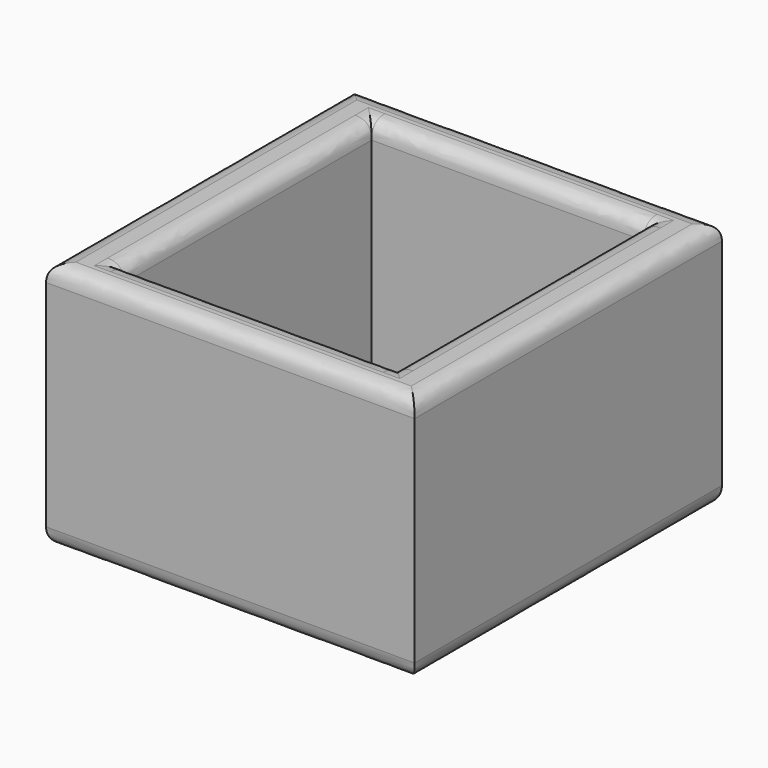
from build123d import *

# Parameters (mm, degrees)
F0_W         = 113.1491363049
F0_H         = 117.9769933224
F1_DEPTH     = 76.2
F2_W         = 83.599075675
F2_H         = 95.0139909983
F3_DEPTH     = 105.1160246134
F4_T1_DEPTH  = 83.599075675
F4_T3_DEPTH  = 95.0139909983
F4_T5_DEPTH  = 138.5491363049
F4_T7_DEPTH  = 143.3769933224
F4_T13_DEPTH = 96.299075675
F4_T17_DEPTH = 107.7139909983
F4_T24_DEPTH = 107.7139909983
F4_T28_DEPTH = 96.299075675
F4_T35_DEPTH = 107.7139909983
F4_T39_DEPTH = 96.299075675
F4_T46_DEPTH = 107.7139909983
F4_T50_DEPTH = 96.299075675
F4_T57_DEPTH = 96.299075675
F4_T61_DEPTH = 107.7139909983
F4_T68_DEPTH = 96.299075675
F4_T72_DEPTH = 107.7139909983
F4_T79_DEPTH = 107.7139909983
F4_T83_DEPTH = 96.299075675
F4_T90_DEPTH = 96.299075675
F4_T94_DEPTH = 107.7139909983


# Not quite as in the source:
# - a fillet or chamfer that OpenCascade refuses, or shapes differently, is made with other operations: its cross-section is extruded or revolved along the edge and cut away or added


with BuildPart() as f1:
    # F0 (on Top) → F1 (new body)
    with BuildSketch(Plane.XY):
        Rectangle(F0_W, F0_H)
    extrude(amount=F1_DEPTH)

    # F2 (on Top) → F3 (cut)
    with BuildSketch(Plane.XY):
        Rectangle(F2_W, F2_H)
    extrude(amount=F3_DEPTH, mode=Mode.SUBTRACT)

    # F4: fillet of radius 5.08 on 16 edges, made by hand

    # F4_s2 → F4_t1 (cut)
    with BuildSketch(Plane.YZ.offset(-41.7995378375)):
        with BuildLine():
            add(Edge.make_bspline(
                [(-52.5869954991, 76.2), (-47.5069954991, 76.2), (-47.5069954991, 71.12)],
                knots=[0, 0, 0, 1, 1, 1], degree=2, weights=[1, 1, 1]))
            Line((-47.5069954991, 71.12), (-47.5069954991, 76.2))
            Line((-47.5069954991, 76.2), (-52.5869954991, 76.2))
        make_face()
        with BuildLine():
            add(Edge.make_bspline(
                [(52.5869954991, 76.2), (47.5069954991, 76.2), (47.5069954991, 71.12)],
                knots=[0, 0, 0, 1, 1, 1], degree=2, weights=[1, 1, 1]))
            Line((47.5069954991, 71.12), (47.5069954991, 76.2))
            Line((47.5069954991, 76.2), (52.5869954991, 76.2))
        make_face()
        with BuildLine():
            add(Edge.make_bspline(
                [(52.5869954991, 0), (47.5069954991, 0), (47.5069954991, 5.08)],
                knots=[0, 0, 0, 1, 1, 1], degree=2, weights=[1, 1, 1]))
            Line((47.5069954991, 5.08), (47.5069954991, 0))
            Line((47.5069954991, 0), (52.5869954991, 0))
        make_face()
        with BuildLine():
            add(Edge.make_bspline(
                [(-52.5869954991, 0), (-47.5069954991, 0), (-47.5069954991, 5.08)],
                knots=[0, 0, 0, 1, 1, 1], degree=2, weights=[1, 1, 1]))
            Line((-47.5069954991, 5.08), (-47.5069954991, 0))
            Line((-47.5069954991, 0), (-52.5869954991, 0))
        make_face()
    extrude(amount=F4_T1_DEPTH, mode=Mode.SUBTRACT)

    # F4_s4 → F4_t3 (cut)
    with BuildSketch(Plane.XZ.offset(-47.5069954991)):
        with BuildLine():
            add(Edge.make_bspline(
                [(-46.8795378375, 76.2), (-41.7995378375, 76.2), (-41.7995378375, 71.12)],
                knots=[0, 0, 0, 1, 1, 1], degree=2, weights=[1, 1, 1]))
            Line((-41.7995378375, 71.12), (-41.7995378375, 76.2))
            Line((-41.7995378375, 76.2), (-46.8795378375, 76.2))
        make_face()
        with BuildLine():
            add(Edge.make_bspline(
                [(46.8795378375, 76.2), (41.7995378375, 76.2), (41.7995378375, 71.12)],
                knots=[0, 0, 0, 1, 1, 1], degree=2, weights=[1, 1, 1]))
            Line((41.7995378375, 71.12), (41.7995378375, 76.2))
            Line((41.7995378375, 76.2), (46.8795378375, 76.2))
        make_face()
        with BuildLine():
            add(Edge.make_bspline(
                [(-46.8795378375, 0), (-41.7995378375, 0), (-41.7995378375, 5.08)],
                knots=[0, 0, 0, 1, 1, 1], degree=2, weights=[1, 1, 1]))
            Line((-41.7995378375, 5.08), (-41.7995378375, 0))
            Line((-41.7995378375, 0), (-46.8795378375, 0))
        make_face()
        with BuildLine():
            add(Edge.make_bspline(
                [(46.8795378375, 0), (41.7995378375, 0), (41.7995378375, 5.08)],
                knots=[0, 0, 0, 1, 1, 1], degree=2, weights=[1, 1, 1]))
            Line((41.7995378375, 5.08), (41.7995378375, 0))
            Line((41.7995378375, 0), (46.8795378375, 0))
        make_face()
    extrude(amount=F4_T3_DEPTH, mode=Mode.SUBTRACT)

    # F4_s6 → F4_t5 (cut)
    with BuildSketch(Plane.YZ.offset(-69.2745681524)):
        with BuildLine():
            add(Edge.make_bspline(
                [(53.9084966612, 76.2), (58.9884966612, 76.2), (58.9884966612, 71.12)],
                knots=[0, 0, 0, 1, 1, 1], degree=2, weights=[1, 1, 1]))
            Line((58.9884966612, 71.12), (58.9884966612, 76.2))
            Line((58.9884966612, 76.2), (53.9084966612, 76.2))
        make_face()
        with BuildLine():
            add(Edge.make_bspline(
                [(-58.9884966612, 71.12), (-58.9884966612, 76.2), (-53.9084966612, 76.2)],
                knots=[0, 0, 0, 1, 1, 1], degree=2, weights=[1, 1, 1]))
            Line((-53.9084966612, 76.2), (-58.9884966612, 76.2))
            Line((-58.9884966612, 76.2), (-58.9884966612, 71.12))
        make_face()
        with BuildLine():
            add(Edge.make_bspline(
                [(-58.9884966612, 5.08), (-58.9884966612, 0), (-53.9084966612, 0)],
                knots=[0, 0, 0, 1, 1, 1], degree=2, weights=[1, 1, 1]))
            Line((-53.9084966612, 0), (-58.9884966612, 0))
            Line((-58.9884966612, 0), (-58.9884966612, 5.08))
        make_face()
        with BuildLine():
            add(Edge.make_bspline(
                [(53.9084966612, 0), (58.9884966612, 0), (58.9884966612, 5.08)],
                knots=[0, 0, 0, 1, 1, 1], degree=2, weights=[1, 1, 1]))
            Line((58.9884966612, 5.08), (58.9884966612, 0))
            Line((58.9884966612, 0), (53.9084966612, 0))
        make_face()
    extrude(amount=F4_T5_DEPTH, mode=Mode.SUBTRACT)

    # F4_s8 → F4_t7 (cut)
    with BuildSketch(Plane.XZ.offset(-71.6884966612)):
        with BuildLine():
            add(Edge.make_bspline(
                [(56.5745681524, 71.12), (56.5745681524, 76.2), (51.4945681524, 76.2)],
                knots=[0, 0, 0, 1, 1, 1], degree=2, weights=[1, 1, 1]))
            Line((51.4945681524, 76.2), (56.5745681524, 76.2))
            Line((56.5745681524, 76.2), (56.5745681524, 71.12))
        make_face()
        with BuildLine():
            add(Edge.make_bspline(
                [(-56.5745681524, 71.12), (-56.5745681524, 76.2), (-51.4945681524, 76.2)],
                knots=[0, 0, 0, 1, 1, 1], degree=2, weights=[1, 1, 1]))
            Line((-51.4945681524, 76.2), (-56.5745681524, 76.2))
            Line((-56.5745681524, 76.2), (-56.5745681524, 71.12))
        make_face()
        with BuildLine():
            add(Edge.make_bspline(
                [(-56.5745681524, 5.08), (-56.5745681524, 0), (-51.4945681524, 0)],
                knots=[0, 0, 0, 1, 1, 1], degree=2, weights=[1, 1, 1]))
            Line((-51.4945681524, 0), (-56.5745681524, 0))
            Line((-56.5745681524, 0), (-56.5745681524, 5.08))
        make_face()
        with BuildLine():
            add(Edge.make_bspline(
                [(56.5745681524, 5.08), (56.5745681524, 0), (51.4945681524, 0)],
                knots=[0, 0, 0, 1, 1, 1], degree=2, weights=[1, 1, 1]))
            Line((51.4945681524, 0), (56.5745681524, 0))
            Line((56.5745681524, 0), (56.5745681524, 5.08))
        make_face()
    extrude(amount=F4_T7_DEPTH, mode=Mode.SUBTRACT)


with BuildPart() as f4_tool11:
    # F4_s12 → F4_t13 (new body)
    with BuildSketch(Plane.YZ.offset(54.4995378375)):
        with BuildLine():
            add(Edge.make_bspline(
                [(-52.5869954991, 76.2), (-47.5069954991, 76.2), (-47.5069954991, 71.12)],
                knots=[0, 0, 0, 1, 1, 1], degree=2, weights=[1, 1, 1]))
            Line((-47.5069954991, 71.12), (-47.5069954991, 76.2))
            Line((-47.5069954991, 76.2), (-52.5869954991, 76.2))
        make_face()
    extrude(amount=-F4_T13_DEPTH)

    split(bisect_by=Plane.YZ.offset(41.7995378375), keep=Keep.TOP)


with BuildPart() as f4_tool15:
    # F4_s16 → F4_t17 (new body)
    with BuildSketch(Plane.XZ.offset(-47.5069954991)):
        with BuildLine():
            add(Edge.make_bspline(
                [(46.8795378375, 76.2), (41.7995378375, 76.2), (41.7995378375, 71.12)],
                knots=[0, 0, 0, 1, 1, 1], degree=2, weights=[1, 1, 1]))
            Line((41.7995378375, 71.12), (41.7995378375, 76.2))
            Line((41.7995378375, 76.2), (46.8795378375, 76.2))
        make_face()
    extrude(amount=F4_T17_DEPTH)

    split(bisect_by=Plane.XZ.offset(47.5069954991), keep=Keep.TOP)


with BuildPart() as f4_tool11_1:
    add(f4_tool11.part)

    # F4_t19: intersect F4_tool15
    add(f4_tool15.part, mode=Mode.INTERSECT)


with BuildPart() as f1_1:
    add(f1.part)

    # F4_t9: cut F4_tool11
    add(f4_tool11_1.part, mode=Mode.SUBTRACT)


with BuildPart() as f4_tool22:
    # F4_s23 → F4_t24 (new body)
    with BuildSketch(Plane.XZ.offset(60.2069954991)):
        with BuildLine():
            add(Edge.make_bspline(
                [(-46.8795378375, 76.2), (-41.7995378375, 76.2), (-41.7995378375, 71.12)],
                knots=[0, 0, 0, 1, 1, 1], degree=2, weights=[1, 1, 1]))
            Line((-41.7995378375, 71.12), (-41.7995378375, 76.2))
            Line((-41.7995378375, 76.2), (-46.8795378375, 76.2))
        make_face()
    extrude(amount=-F4_T24_DEPTH)

    split(bisect_by=Plane.XZ.offset(47.5069954991), keep=Keep.TOP)


with BuildPart() as f4_tool26:
    # F4_s27 → F4_t28 (new body)
    with BuildSketch(Plane.YZ.offset(41.7995378375)):
        with BuildLine():
            add(Edge.make_bspline(
                [(-52.5869954991, 76.2), (-47.5069954991, 76.2), (-47.5069954991, 71.12)],
                knots=[0, 0, 0, 1, 1, 1], degree=2, weights=[1, 1, 1]))
            Line((-47.5069954991, 71.12), (-47.5069954991, 76.2))
            Line((-47.5069954991, 76.2), (-52.5869954991, 76.2))
        make_face()
    extrude(amount=-F4_T28_DEPTH)

    split(bisect_by=Plane.YZ.offset(-41.7995378375), keep=Keep.BOTTOM)


with BuildPart() as f4_tool22_1:
    add(f4_tool22.part)

    # F4_t30: intersect F4_tool26
    add(f4_tool26.part, mode=Mode.INTERSECT)


with BuildPart() as f1_2:
    add(f1_1.part)

    # F4_t20: cut F4_tool22
    add(f4_tool22_1.part, mode=Mode.SUBTRACT)


with BuildPart() as f4_tool33:
    # F4_s34 → F4_t35 (new body)
    with BuildSketch(Plane.XZ.offset(47.5069954991)):
        with BuildLine():
            add(Edge.make_bspline(
                [(-46.8795378375, 76.2), (-41.7995378375, 76.2), (-41.7995378375, 71.12)],
                knots=[0, 0, 0, 1, 1, 1], degree=2, weights=[1, 1, 1]))
            Line((-41.7995378375, 71.12), (-41.7995378375, 76.2))
            Line((-41.7995378375, 76.2), (-46.8795378375, 76.2))
        make_face()
    extrude(amount=-F4_T35_DEPTH)

    split(bisect_by=Plane.XZ.offset(-47.5069954991), keep=Keep.BOTTOM)


with BuildPart() as f4_tool37:
    # F4_s38 → F4_t39 (new body)
    with BuildSketch(Plane.YZ.offset(-54.4995378375)):
        with BuildLine():
            add(Edge.make_bspline(
                [(52.5869954991, 76.2), (47.5069954991, 76.2), (47.5069954991, 71.12)],
                knots=[0, 0, 0, 1, 1, 1], degree=2, weights=[1, 1, 1]))
            Line((47.5069954991, 71.12), (47.5069954991, 76.2))
            Line((47.5069954991, 76.2), (52.5869954991, 76.2))
        make_face()
    extrude(amount=F4_T39_DEPTH)

    split(bisect_by=Plane.YZ.offset(-41.7995378375), keep=Keep.BOTTOM)


with BuildPart() as f4_tool33_1:
    add(f4_tool33.part)

    # F4_t41: intersect F4_tool37
    add(f4_tool37.part, mode=Mode.INTERSECT)


with BuildPart() as f1_3:
    add(f1_2.part)

    # F4_t31: cut F4_tool33
    add(f4_tool33_1.part, mode=Mode.SUBTRACT)


with BuildPart() as f4_tool44:
    # F4_s45 → F4_t46 (new body)
    with BuildSketch(Plane.XZ.offset(-60.2069954991)):
        with BuildLine():
            add(Edge.make_bspline(
                [(46.8795378375, 76.2), (41.7995378375, 76.2), (41.7995378375, 71.12)],
                knots=[0, 0, 0, 1, 1, 1], degree=2, weights=[1, 1, 1]))
            Line((41.7995378375, 71.12), (41.7995378375, 76.2))
            Line((41.7995378375, 76.2), (46.8795378375, 76.2))
        make_face()
    extrude(amount=F4_T46_DEPTH)

    split(bisect_by=Plane.XZ.offset(-47.5069954991), keep=Keep.BOTTOM)


with BuildPart() as f4_tool48:
    # F4_s49 → F4_t50 (new body)
    with BuildSketch(Plane.YZ.offset(-41.7995378375)):
        with BuildLine():
            add(Edge.make_bspline(
                [(52.5869954991, 76.2), (47.5069954991, 76.2), (47.5069954991, 71.12)],
                knots=[0, 0, 0, 1, 1, 1], degree=2, weights=[1, 1, 1]))
            Line((47.5069954991, 71.12), (47.5069954991, 76.2))
            Line((47.5069954991, 76.2), (52.5869954991, 76.2))
        make_face()
    extrude(amount=F4_T50_DEPTH)

    split(bisect_by=Plane.YZ.offset(41.7995378375), keep=Keep.TOP)


with BuildPart() as f4_tool44_1:
    add(f4_tool44.part)

    # F4_t52: intersect F4_tool48
    add(f4_tool48.part, mode=Mode.INTERSECT)


with BuildPart() as f1_4:
    add(f1_3.part)

    # F4_t42: cut F4_tool44
    add(f4_tool44_1.part, mode=Mode.SUBTRACT)


with BuildPart() as f4_tool55:
    # F4_s56 → F4_t57 (new body)
    with BuildSketch(Plane.YZ.offset(54.4995378375)):
        with BuildLine():
            add(Edge.make_bspline(
                [(52.5869954991, 0), (47.5069954991, 0), (47.5069954991, 5.08)],
                knots=[0, 0, 0, 1, 1, 1], degree=2, weights=[1, 1, 1]))
            Line((47.5069954991, 5.08), (47.5069954991, 0))
            Line((47.5069954991, 0), (52.5869954991, 0))
        make_face()
    extrude(amount=-F4_T57_DEPTH)

    split(bisect_by=Plane.YZ.offset(41.7995378375), keep=Keep.TOP)


with BuildPart() as f4_tool59:
    # F4_s60 → F4_t61 (new body)
    with BuildSketch(Plane.XZ.offset(47.5069954991)):
        with BuildLine():
            add(Edge.make_bspline(
                [(46.8795378375, 0), (41.7995378375, 0), (41.7995378375, 5.08)],
                knots=[0, 0, 0, 1, 1, 1], degree=2, weights=[1, 1, 1]))
            Line((41.7995378375, 5.08), (41.7995378375, 0))
            Line((41.7995378375, 0), (46.8795378375, 0))
        make_face()
    extrude(amount=-F4_T61_DEPTH)

    split(bisect_by=Plane.XZ.offset(-47.5069954991), keep=Keep.BOTTOM)


with BuildPart() as f4_tool55_1:
    add(f4_tool55.part)

    # F4_t63: intersect F4_tool59
    add(f4_tool59.part, mode=Mode.INTERSECT)


with BuildPart() as f1_5:
    add(f1_4.part)

    # F4_t53: cut F4_tool55
    add(f4_tool55_1.part, mode=Mode.SUBTRACT)


with BuildPart() as f4_tool66:
    # F4_s67 → F4_t68 (new body)
    with BuildSketch(Plane.YZ.offset(41.7995378375)):
        with BuildLine():
            add(Edge.make_bspline(
                [(52.5869954991, 0), (47.5069954991, 0), (47.5069954991, 5.08)],
                knots=[0, 0, 0, 1, 1, 1], degree=2, weights=[1, 1, 1]))
            Line((47.5069954991, 5.08), (47.5069954991, 0))
            Line((47.5069954991, 0), (52.5869954991, 0))
        make_face()
    extrude(amount=-F4_T68_DEPTH)

    split(bisect_by=Plane.YZ.offset(-41.7995378375), keep=Keep.BOTTOM)


with BuildPart() as f4_tool70:
    # F4_s71 → F4_t72 (new body)
    with BuildSketch(Plane.XZ.offset(-60.2069954991)):
        with BuildLine():
            add(Edge.make_bspline(
                [(-46.8795378375, 0), (-41.7995378375, 0), (-41.7995378375, 5.08)],
                knots=[0, 0, 0, 1, 1, 1], degree=2, weights=[1, 1, 1]))
            Line((-41.7995378375, 5.08), (-41.7995378375, 0))
            Line((-41.7995378375, 0), (-46.8795378375, 0))
        make_face()
    extrude(amount=F4_T72_DEPTH)

    split(bisect_by=Plane.XZ.offset(-47.5069954991), keep=Keep.BOTTOM)


with BuildPart() as f4_tool66_1:
    add(f4_tool66.part)

    # F4_t74: intersect F4_tool70
    add(f4_tool70.part, mode=Mode.INTERSECT)


with BuildPart() as f1_6:
    add(f1_5.part)

    # F4_t64: cut F4_tool66
    add(f4_tool66_1.part, mode=Mode.SUBTRACT)


with BuildPart() as f4_tool77:
    # F4_s78 → F4_t79 (new body)
    with BuildSketch(Plane.XZ.offset(-47.5069954991)):
        with BuildLine():
            add(Edge.make_bspline(
                [(-46.8795378375, 0), (-41.7995378375, 0), (-41.7995378375, 5.08)],
                knots=[0, 0, 0, 1, 1, 1], degree=2, weights=[1, 1, 1]))
            Line((-41.7995378375, 5.08), (-41.7995378375, 0))
            Line((-41.7995378375, 0), (-46.8795378375, 0))
        make_face()
    extrude(amount=F4_T79_DEPTH)

    split(bisect_by=Plane.XZ.offset(47.5069954991), keep=Keep.TOP)


with BuildPart() as f4_tool81:
    # F4_s82 → F4_t83 (new body)
    with BuildSketch(Plane.YZ.offset(-54.4995378375)):
        with BuildLine():
            add(Edge.make_bspline(
                [(-52.5869954991, 0), (-47.5069954991, 0), (-47.5069954991, 5.08)],
                knots=[0, 0, 0, 1, 1, 1], degree=2, weights=[1, 1, 1]))
            Line((-47.5069954991, 5.08), (-47.5069954991, 0))
            Line((-47.5069954991, 0), (-52.5869954991, 0))
        make_face()
    extrude(amount=F4_T83_DEPTH)

    split(bisect_by=Plane.YZ.offset(-41.7995378375), keep=Keep.BOTTOM)


with BuildPart() as f4_tool77_1:
    add(f4_tool77.part)

    # F4_t85: intersect F4_tool81
    add(f4_tool81.part, mode=Mode.INTERSECT)


with BuildPart() as f1_7:
    add(f1_6.part)

    # F4_t75: cut F4_tool77
    add(f4_tool77_1.part, mode=Mode.SUBTRACT)


with BuildPart() as f4_tool88:
    # F4_s89 → F4_t90 (new body)
    with BuildSketch(Plane.YZ.offset(-41.7995378375)):
        with BuildLine():
            add(Edge.make_bspline(
                [(-52.5869954991, 0), (-47.5069954991, 0), (-47.5069954991, 5.08)],
                knots=[0, 0, 0, 1, 1, 1], degree=2, weights=[1, 1, 1]))
            Line((-47.5069954991, 5.08), (-47.5069954991, 0))
            Line((-47.5069954991, 0), (-52.5869954991, 0))
        make_face()
    extrude(amount=F4_T90_DEPTH)

    split(bisect_by=Plane.YZ.offset(41.7995378375), keep=Keep.TOP)


with BuildPart() as f4_tool92:
    # F4_s93 → F4_t94 (new body)
    with BuildSketch(Plane.XZ.offset(60.2069954991)):
        with BuildLine():
            add(Edge.make_bspline(
                [(46.8795378375, 0), (41.7995378375, 0), (41.7995378375, 5.08)],
                knots=[0, 0, 0, 1, 1, 1], degree=2, weights=[1, 1, 1]))
            Line((41.7995378375, 5.08), (41.7995378375, 0))
            Line((41.7995378375, 0), (46.8795378375, 0))
        make_face()
    extrude(amount=-F4_T94_DEPTH)

    split(bisect_by=Plane.XZ.offset(47.5069954991), keep=Keep.TOP)


with BuildPart() as f4_tool88_1:
    add(f4_tool88.part)

    # F4_t96: intersect F4_tool92
    add(f4_tool92.part, mode=Mode.INTERSECT)


with BuildPart() as f1_8:
    add(f1_7.part)

    # F4_t86: cut F4_tool88
    add(f4_tool88_1.part, mode=Mode.SUBTRACT)


solid = f1_8.part
